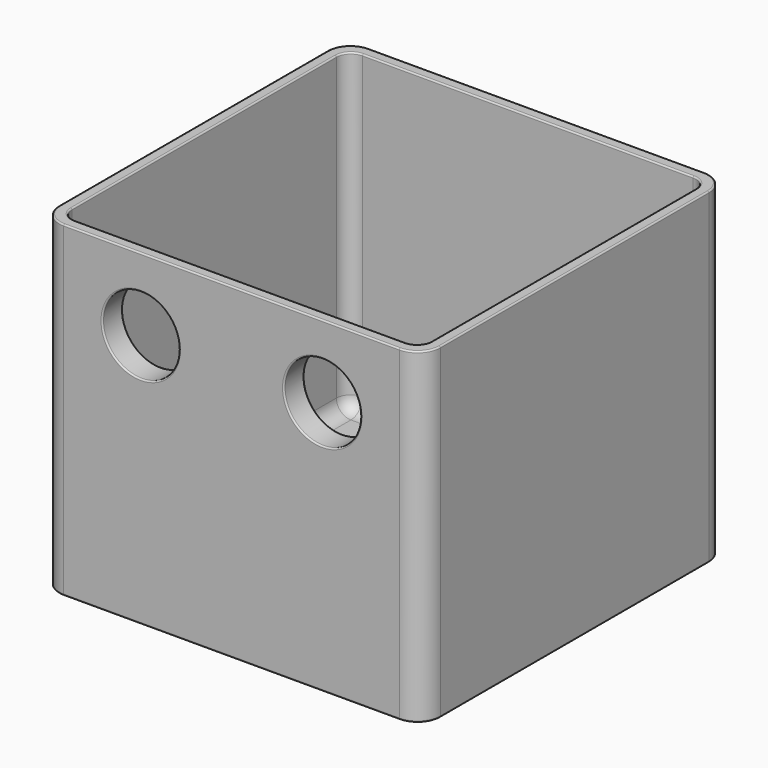
from build123d import *

# Parameters (mm, degrees)
F0_W     = 133.35
F0_H     = 133.35
F1_DEPTH = 114.3
F3_W     = 125.73
F3_H     = 125.73
F4_DEPTH = 110.49
F5_R     = 17.8435
F5_R_2   = 13.3985
F6_DEPTH = 8.89
F7_DEPTH = 3.81
F8_R     = 5.08
F9_R     = 8.001
F10_R    = 0.508
F11_R    = 2.54


# Not quite as in the source:
# - two fillets or chamfers of one size are made in one step


with BuildPart() as f1:
    # F0 (on Top) → F1 (new body)
    with BuildSketch(Plane.XY):
        Rectangle(F0_W, F0_H)
    extrude(amount=F1_DEPTH)

    # F3 (on offset) → F4 (cut, through all)
    with BuildSketch(Plane.XY.offset(3.81)):
        Rectangle(F3_W, F3_H)
    extrude(amount=F4_DEPTH, mode=Mode.SUBTRACT)

    # F5 (on face) → F6 (join)
    with BuildSketch(Plane.XZ.offset(66.675)):
        with Locations((-31.75, 88.9)):
            Circle(F5_R)
        with Locations((-31.75, 88.9)):
            Circle(F5_R_2, mode=Mode.SUBTRACT)
        with Locations((31.75, 88.9)):
            Circle(F5_R)
        with Locations((31.75, 88.9)):
            Circle(F5_R_2, mode=Mode.SUBTRACT)
    extrude(amount=-F6_DEPTH)

    # F5 (on face) → F7 (cut, through all)
    with BuildSketch(Plane.XZ.offset(66.675)):
        with Locations((-31.75, 88.9)):
            Circle(F5_R_2)
        with Locations((31.75, 88.9)):
            Circle(F5_R_2)
    extrude(amount=-F7_DEPTH, mode=Mode.SUBTRACT)

    # F8
    f8_edges = [f1.edges().sort_by_distance(p)[0] for p in [
        (-62.865, 0, 3.81),
        (0, 62.865, 3.81),
        (62.865, 0, 3.81),
        (0, -62.865, 3.81),
        (62.865, -62.865, 59.055),
        (-62.865, -62.865, 59.055),
        (-62.865, 62.865, 59.055),
        (62.865, 62.865, 59.055),
    ]]
    fillet(f8_edges, radius=F8_R)

    # F9
    f9_edges = [f1.edges().sort_by_distance(p)[0] for p in [
        (-66.675, 66.675, 57.15),
        (66.675, 66.675, 57.15),
        (-66.675, -66.675, 57.15),
        (66.675, -66.675, 57.15),
    ]]
    fillet(f9_edges, radius=F9_R)

    # F10
    f10_edges = [f1.edges().sort_by_distance(p)[0] for p in [
        (-45.1485, -66.675, 88.9),
        (18.3515, -66.675, 88.9),
        (-45.1485, -57.785, 88.9),
        (18.3515, -57.785, 88.9),
        (66.675, 0, 114.3),
        (64.331561, -64.331561, 114.3),
        (64.331561, 64.331561, 114.3),
        (0, -66.675, 114.3),
        (0, 66.675, 114.3),
        (-64.331561, -64.331561, 114.3),
        (-64.331561, 64.331561, 114.3),
        (-66.675, 0, 114.3),
        (62.865, 0, 114.3),
        (61.377102, -61.377102, 114.3),
        (61.377102, 61.377102, 114.3),
        (0, -62.865, 114.3),
        (0, 62.865, 114.3),
        (-61.377102, -61.377102, 114.3),
        (-61.377102, 61.377102, 114.3),
        (-62.865, 0, 114.3),
        (66.675, 0, 0),
        (64.331561, -64.331561, 0),
        (64.331561, 64.331561, 0),
        (0, -66.675, 0),
        (0, 66.675, 0),
        (-64.331561, -64.331561, 0),
        (-64.331561, 64.331561, 0),
        (-66.675, 0, 0),
        (-49.5935, -57.785, 88.9),
    ]]
    fillet(f10_edges, radius=F10_R)

    # F11
    f11_edges = [f1.edges().sort_by_distance(p)[0] for p in [
        (-49.5935, -62.865, 88.9),
        (13.9065, -62.865, 88.9),
    ]]
    fillet(f11_edges, radius=F11_R)


solid = f1.part
